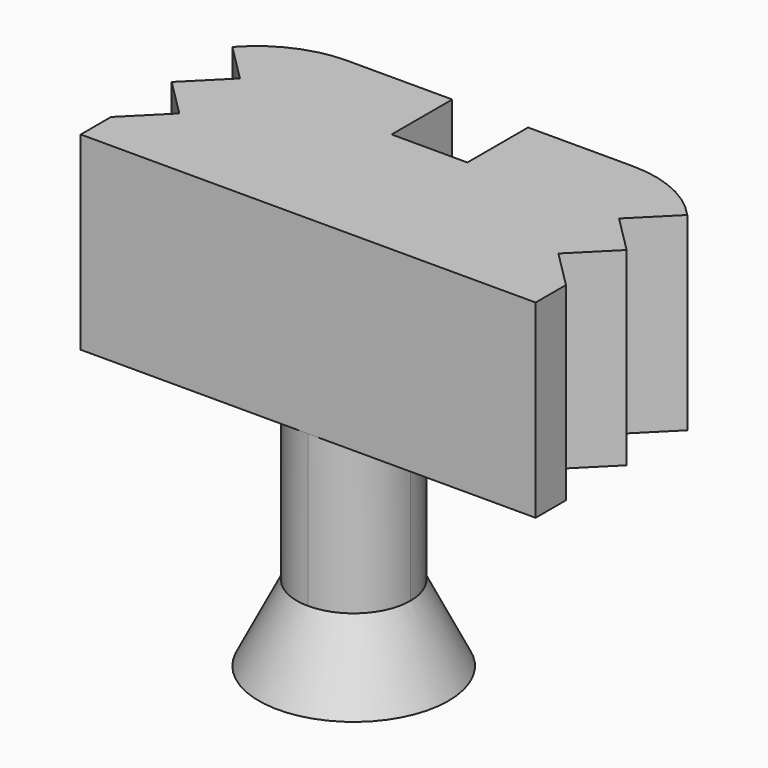
from build123d import *

# Parameters (mm, degrees)
F0_W        = 2
F0_H        = 2
F1_DEPTH    = 5
F2_W        = 3
F2_H        = 3
F3_DEPTH    = 4
F4_R        = 1.49999
F5_W        = 2
F5_H        = 2
F6_DEPTH    = 5
F8_DEPTH    = 9.001
F9_T1_DEPTH = 16.1803398875
F10_R       = 1.5
F12_R       = 2.5


# Not quite as in the source:
# - a fillet or chamfer that OpenCascade refuses, or shapes differently, is made with other operations: its cross-section is extruded or revolved along the edge and cut away or added
# - a fillet or chamfer is up to 0.001 mm smaller than in the source, because OpenCascade refuses the exact size


with BuildPart() as f1:
    # F0 (on Top) → F1 (new body)
    with BuildSketch(Plane.XY):
        Polygon((-6, -3), (6, -3), (6, 3), (1, 3), (1, 1), (-1, 1), (-1, 3), (-6, 3), align=None)
        with Locations((0, 2)):
            Rectangle(F0_W, F0_H)
    extrude(amount=F1_DEPTH)

    # F2 (on face) → F3 (join)
    with BuildSketch(Plane(origin=(0, 0, 0), x_dir=(1, 0, 0), z_dir=(0, 0, -1))):
        with Locations((0, 1.5)):
            Rectangle(F2_W, F2_H)
    extrude(amount=F3_DEPTH)

    # F4 (radius 1.5 in the source; OpenCascade refuses exactly that, so slightly less here)
    f4_edges = [f1.edges().sort_by_distance(p)[0] for p in [
        (-1.5, 0, -2),
        (1.5, 0, -2),
        (-1.5, -3, -2),
        (1.5, -3, -2),
    ]]
    fillet(f4_edges, radius=F4_R)

    # F5 (on face) → F6 (cut, through all)
    with BuildSketch(Plane.XY.offset(5)):
        with Locations((0, 2)):
            Rectangle(F5_W, F5_H)
    extrude(amount=-F6_DEPTH, mode=Mode.SUBTRACT)

    # F7 (on face) → F8 (cut, through all)
    with BuildSketch(Plane.XY.offset(5)):
        Polygon((-5, 1), (-6, 2), (-6, 0), align=None)
        Polygon((-5, -1), (-6, 0), (-6, -2), align=None)
        Polygon((6, -2), (6, 0), (5, -1), align=None)
        Polygon((6, 0), (6, 2), (5, 1), align=None)
    extrude(amount=-F8_DEPTH, mode=Mode.SUBTRACT)

    # F9: fillet of radius 3 on 2 edges, made by hand

    # F9_s2 → F9_t1 (cut)
    with BuildSketch(Plane.XY.offset(-5.5901699437)):
        with BuildLine():
            ThreePointArc((-6, 2), (-4.9886768939, 2.7386127875), (-3.7639320225, 3))
            Line((-3.7639320225, 3), (-6, 3))
            Line((-6, 3), (-6, 2))
        make_face()
        with BuildLine():
            ThreePointArc((3.7639320225, 3), (4.9886768939, 2.7386127875), (6, 2))
            Line((6, 2), (6, 3))
            Line((6, 3), (3.7639320225, 3))
        make_face()
    extrude(amount=F9_T1_DEPTH, mode=Mode.SUBTRACT)

    # F10 (on face) → F13 section 0
    with BuildSketch(Plane(origin=(0, 0, -4), x_dir=(1, 0, 0), z_dir=(0, 0, -1))):
        with Locations((0, 1.5)):
            Circle(F10_R)
    # F12 (on offset) → F13 section 1
    with BuildSketch(Plane(origin=(0, 0, -6), x_dir=(1, 0, 0), z_dir=(0, 0, -1))):
        with Locations((0, 1.5)):
            Circle(F12_R)
    loft()


solid = f1.part
